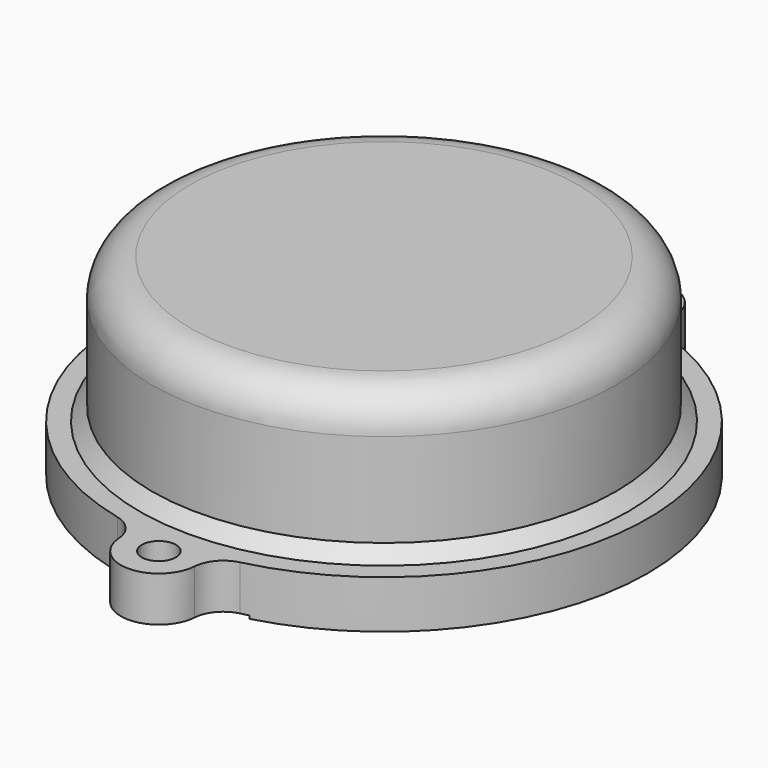
from build123d import *

# Parameters (mm, degrees)
F2_R        = 2.8448
F3_DEPTH    = 7.5184
F2_R_2      = 6.35
F4_DEPTH    = 7.5184
F5_R        = 5.08
F6_T1_DEPTH = 7.5184
F9_DEPTH    = 0.508


# Not quite as in the source:
# - a fillet or chamfer that OpenCascade refuses, or shapes differently, is made with other operations: its cross-section is extruded or revolved along the edge and cut away or added
# - two fillets or chamfers of one size are made in one step


with BuildPart() as f1:
    # F0 (on Front) → F1 (revolve)
    with BuildSketch(Plane.XZ):
        with BuildLine():
            Line((32.385, 31.75), (0, 31.75))
            Line((0, 31.75), (0, 28.575))
            Line((0, 28.575), (32.4854701757, 28.575))
            Line((32.4854701757, 28.575), (35.56, 25.49819462))
            Line((35.56, 25.49819462), (35.56, 8.8277412578))
            Line((35.56, 8.8277412578), (39.5224, 4.572))
            Line((39.5224, 4.572), (39.5224, 0))
            Line((39.5224, 0), (43.053, 0))
            Line((43.053, 0), (43.053, -0.508))
            Line((43.053, -0.508), (44.069, -0.508))
            Line((44.069, -0.508), (44.069, 7.5184))
            Line((44.069, 7.5184), (40.8266418362, 7.5184))
            Line((40.8266418362, 7.5184), (38.735, 9.7710676491))
            Line((38.735, 9.7710676491), (38.735, 25.4))
            ThreePointArc((38.735, 25.4), (36.8751280605, 29.8901280605), (32.385, 31.75))
        make_face()
    revolve(axis=Axis((0, 0, 30.1625), (0, 0, 1)))

    # F2 (on face) → F3 (join)
    with BuildSketch(Plane(origin=(0, 0, 0), x_dir=(1, 0, 0), z_dir=(0, 0, -1))):
        with BuildLine():
            ThreePointArc((4.7616218936, 42.7888743243), (5.939646413, 44.7443151405), (6.35, 46.99))
            ThreePointArc((6.35, 46.99), (-2.2456848595, 52.929646413), (-4.7616218936, 42.7888743243))
            ThreePointArc((-4.7616218936, 42.7888743243), (0, 43.053), (4.7616218936, 42.7888743243))
        make_face()
        with Locations((0, 46.99)):
            Circle(F2_R, mode=Mode.SUBTRACT)
    extrude(amount=-F3_DEPTH)

    # F2 (on face) → F4 (join)
    with BuildSketch(Plane(origin=(0, 0, 0), x_dir=(1, 0, 0), z_dir=(0, 0, -1))):
        with Locations((0, 46.99)):
            Circle(F2_R_2)
        with Locations((0, 46.99)):
            Circle(F2_R, mode=Mode.SUBTRACT)
        with Locations((4.699, -46.7544596696)):
            Circle(F2_R_2)
        with Locations((4.699, -46.7544596696)):
            Circle(F2_R, mode=Mode.SUBTRACT)
    extrude(amount=-F4_DEPTH)

    # F5
    f5_edges = [f1.edges().sort_by_distance(p)[0] for p in [
        (9.795498, 42.966557, 3.7592),
        (-1.049351, 44.056505, 3.7592),
    ]]
    fillet(f5_edges, radius=F5_R)

    # F6: fillet of radius 5.08 on 2 edges, made by hand

    # F6_s2 → F6_t1 (join)
    with BuildSketch(Plane.XY):
        with BuildLine():
            ThreePointArc((10.2222959919, -42.8670202563), (7.5289917798, -44.5196041815), (6.3336992457, -47.444701952))
            ThreePointArc((6.3336992457, -47.444701952), (6.1774395627, -45.5197141608), (5.4497416206, -43.7307337838))
            ThreePointArc((5.4497416206, -43.7307337838), (7.8479099763, -43.3645831296), (10.2222959919, -42.8670202563))
        make_face()
        with BuildLine():
            ThreePointArc((-10.2222959919, -42.8670202563), (-7.5289917798, -44.5196041815), (-6.3336992457, -47.444701952))
            ThreePointArc((-6.3336992457, -47.444701952), (-6.1774395627, -45.5197141608), (-5.4497416206, -43.7307337838))
            ThreePointArc((-5.4497416206, -43.7307337838), (-7.8479099763, -43.3645831296), (-10.2222959919, -42.8670202563))
        make_face()
    extrude(amount=F6_T1_DEPTH)

    # F8 (on face) → F9 (cut)
    with BuildSketch(Plane(origin=(0, 0, 0), x_dir=(1, 0, 0), z_dir=(0, 0, -1))):
        with BuildLine():
            Line((11.2232032022, 41.5248573346), (11.5476018718, 42.6009083999))
            ThreePointArc((11.5476018718, 42.6009083999), (0.1217283712, 44.1331880413), (-11.3123981282, 42.6637604833))
            Line((-11.3123981282, 42.6637604833), (-10.9422300011, 41.5995270014))
            ThreePointArc((-10.9422300011, 41.5995270014), (0.145362907, 43.0097069155), (11.2232032022, 41.5248573346))
        make_face()
        with BuildLine():
            Line((-7.2390749119, -42.3223562539), (-7.4246343474, -43.5135134363))
            ThreePointArc((-7.4246343474, -43.5135134363), (4.1004463869, -43.9625847646), (15.3315616772, -41.3374751806))
            Line((15.3315616772, -41.3374751806), (14.8499479477, -40.2801455114))
            ThreePointArc((14.8499479477, -40.2801455114), (3.9400511762, -42.757274104), (-7.2390749119, -42.3223562539))
        make_face()
    extrude(amount=F9_DEPTH, mode=Mode.SUBTRACT)


solid = f1.part
